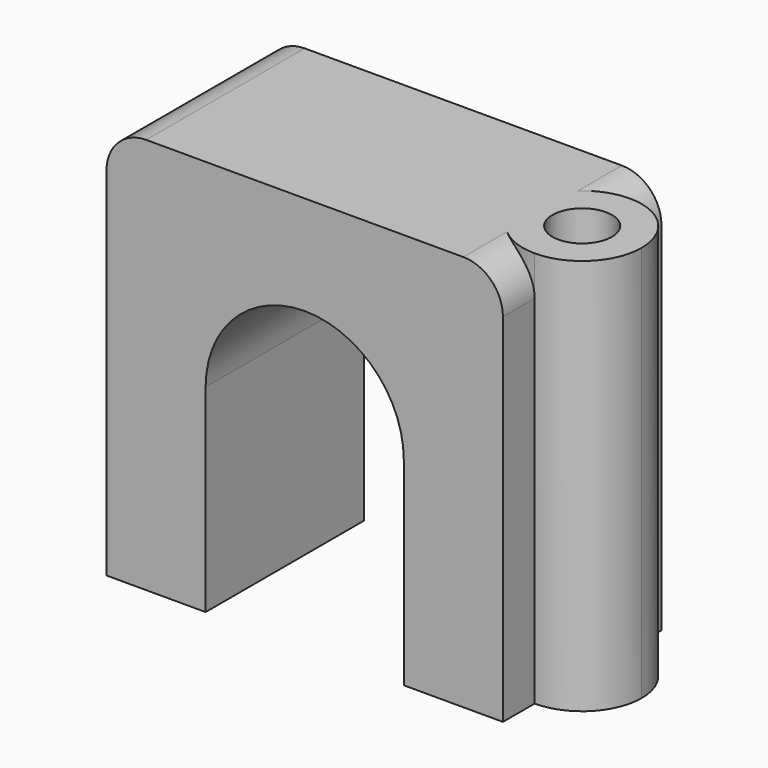
from build123d import *

# Parameters (mm, degrees)
F1_DEPTH     = 50.8
F3_DEPTH     = 25.4
F4_T1_DEPTH  = 50.8
F4_T6_DEPTH  = 30.48
F4_S7_R      = 7.62
F4_T8_DEPTH  = 17
F4_T12_DEPTH = 30.48
F4_S13_R     = 7.62
F4_T14_DEPTH = 17
F6_D         = 7.62


# Not quite as in the source:
# - a fillet or chamfer that OpenCascade refuses, or shapes differently, is made with other operations: its cross-section is extruded or revolved along the edge and cut away or added


with BuildPart() as f1:
    # F0 (on Top) → F1 (new body)
    with BuildSketch(Plane.XY):
        with BuildLine():
            Line((0, 25.4), (0, 0))
            Line((0, 0), (50.8, 0))
            Line((50.8, 0), (50.8, 5.08))
            ThreePointArc((50.8, 5.08), (43.18, 12.7), (50.8, 20.32))
            Line((50.8, 20.32), (50.8, 25.4))
            Line((50.8, 25.4), (0, 25.4))
        make_face()
        with BuildLine():
            Line((50.8, 20.32), (50.8, 5.08))
            ThreePointArc((50.8, 5.08), (56.1881536726, 7.3118463274), (58.42, 12.7))
            ThreePointArc((58.42, 12.7), (56.1881536726, 18.0881536726), (50.8, 20.32))
        make_face()
        with BuildLine():
            ThreePointArc((50.8, 20.32), (43.18, 12.7), (50.8, 5.08))
            Line((50.8, 5.08), (50.8, 20.32))
        make_face()
    extrude(amount=F1_DEPTH)

    # F2 (on face) → F3 (cut)
    with BuildSketch(Plane.XZ):
        with BuildLine():
            ThreePointArc((38.1, 25.4), (25.4, 38.1), (12.7, 25.4))
            Line((12.7, 25.4), (38.1, 25.4))
        make_face()
        with BuildLine():
            Line((38.1, 25.4), (12.7, 25.4))
            ThreePointArc((12.7, 25.4), (25.4, 12.7), (38.1, 25.4))
        make_face()
        with BuildLine():
            Line((12.7, 25.4), (12.7, 0))
            Line((12.7, 0), (38.1, 0))
            Line((38.1, 0), (38.1, 25.4))
            ThreePointArc((38.1, 25.4), (25.4, 12.7), (12.7, 25.4))
        make_face()
    extrude(amount=-F3_DEPTH, mode=Mode.SUBTRACT)

    # F4: fillet of radius 5.08 on 3 edges, made by hand

    # F4_s2 → F4_t1 (cut)
    with BuildSketch(Plane.XZ.offset(-38.1)):
        with BuildLine():
            ThreePointArc((0, 45.72), (1.4878975516, 49.3121024484), (5.08, 50.8))
            Line((5.08, 50.8), (0, 50.8))
            Line((0, 50.8), (0, 45.72))
        make_face()
    extrude(amount=F4_T1_DEPTH, mode=Mode.SUBTRACT)


with BuildPart() as f4_tool4:
    # F4_s5 → F4_t6 (new body)
    with BuildSketch(Plane.XZ.offset(12.7)):
        with BuildLine():
            ThreePointArc((45.72, 50.8), (49.3121024484, 49.3121024484), (50.8, 45.72))
            Line((50.8, 45.72), (50.8, 50.8))
            Line((50.8, 50.8), (45.72, 50.8))
        make_face()
    extrude(amount=-F4_T6_DEPTH)

    # F4_s7 → F4_t8 (cut, symmetric)
    with BuildSketch(Plane.XY.offset(48.3)):
        with Locations((50.8, 12.7)):
            Circle(F4_S7_R)
    extrude(amount=F4_T8_DEPTH, both=True, mode=Mode.SUBTRACT)


with BuildPart() as f1_1:
    add(f1.part)

    # F4_t3: cut F4_tool4
    add(f4_tool4.part, mode=Mode.SUBTRACT)


with BuildPart() as f4_tool10:
    # F4_s11 → F4_t12 (new body)
    with BuildSketch(Plane.XZ.offset(-7.62)):
        with BuildLine():
            ThreePointArc((45.72, 50.8), (49.3121024484, 49.3121024484), (50.8, 45.72))
            Line((50.8, 45.72), (50.8, 50.8))
            Line((50.8, 50.8), (45.72, 50.8))
        make_face()
    extrude(amount=-F4_T12_DEPTH)

    # F4_s13 → F4_t14 (cut, symmetric)
    with BuildSketch(Plane.XY.offset(48.3)):
        with Locations((50.8, 12.7)):
            Circle(F4_S13_R)
    extrude(amount=F4_T14_DEPTH, both=True, mode=Mode.SUBTRACT)


with BuildPart() as f1_2:
    add(f1_1.part)

    # F4_t9: cut F4_tool10
    add(f4_tool10.part, mode=Mode.SUBTRACT)

    # F6 (through all)
    with Locations(Plane.XY.offset(50.8)):
        with Locations((50.8, 12.7)):
            Hole(F6_D / 2)


solid = f1_2.part
